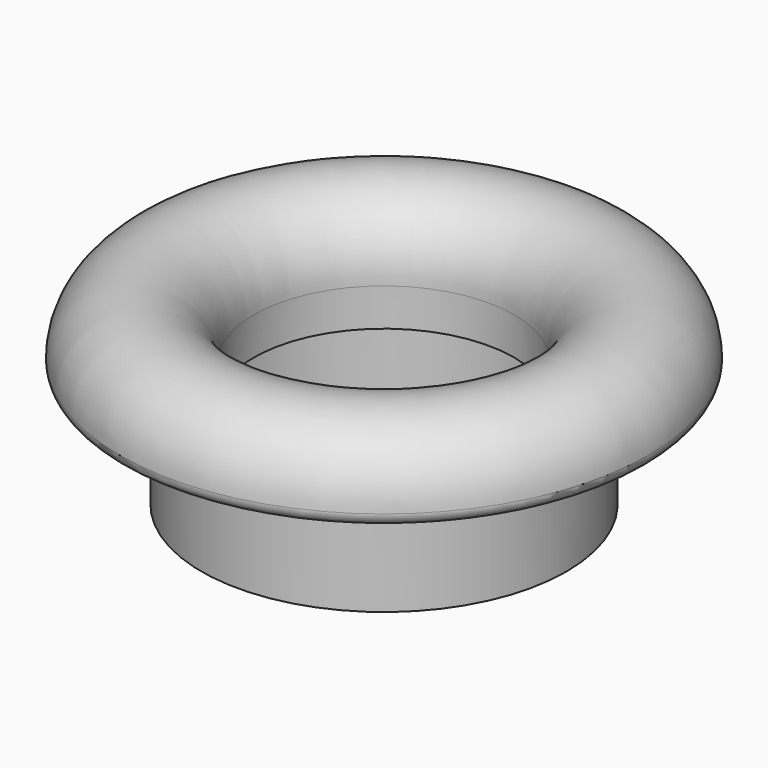
from build123d import *

# Parameters (mm, degrees)
F0_R    = 0.8279940084
F2_SIZE = 1


with BuildPart() as f1:
    # F0 (on Front) → F1 (revolve)
    with BuildSketch(Plane.XZ):
        with Locations((9.5469448715, 20.0060550123)):
            Circle(F0_R)
    revolve(axis=Axis((-15, 0, 28.4551028162), (0, 0, 1)))


with BuildPart() as f1b:
    # F0 (on Front) → F1, piece 2 (revolve)
    with BuildSketch(Plane.XZ):
        with BuildLine():
            ThreePointArc((15.3768501777, 17.9522678642), (7.4242930295, 25.6183157406), (0, 17.4396038463))
            Line((0, 17.4396038463), (0, 13.1062809378))
            Line((0, 13.1062809378), (2.9998879926, 13.1322045127))
            Line((2.9998879926, 13.1322045127), (2.9998879926, 3.1322045127))
            Line((2.9998879926, 3.1322045127), (5.9998879926, 3.1322045127))
            Line((5.9998879926, 3.1322045127), (5.9998879926, 13.1322045127))
            Line((5.9998879926, 13.1322045127), (3.0018545765, 17.5240865694))
            ThreePointArc((3.0018545765, 17.5240865694), (7.4715065543, 22.6179260851), (12.3768670762, 17.9421985519))
            ThreePointArc((12.3768670762, 17.9421985519), (13.8818932831, 16.4472416573), (15.3768501777, 17.9522678642))
        make_face()
        with BuildLine():
            Line((0, 17.4396038463), (0, 18.1062809378))
            Line((0, 18.1062809378), (0.006442766, 17.6866691129))
            Line((0.006442766, 17.6866691129), (0.0128855321, 17.267057288))
            ThreePointArc((0.0128855321, 17.267057288), (0.0059578458, 17.353294354), (0, 17.4396038463))
        make_face(mode=Mode.SUBTRACT)
        with BuildLine():
            Line((0.006442766, 17.6866691129), (0, 18.1062809378))
            Line((0, 18.1062809378), (0, 17.4396038463))
            ThreePointArc((0, 17.4396038463), (0.0059578458, 17.353294354), (0.0128855321, 17.267057288))
            Line((0.0128855321, 17.267057288), (0.006442766, 17.6866691129))
        make_face()
    revolve(axis=Axis((-15, 0, 28.4551028162), (0, 0, 1)))

    # F2
    f2_edges = [f1b.edges().sort_by_distance(p)[0] for p in [
        (-32.999888, 0, 3.132205),
    ]]
    chamfer(f2_edges, length=F2_SIZE)


solid = Compound([f1.part, f1b.part])
